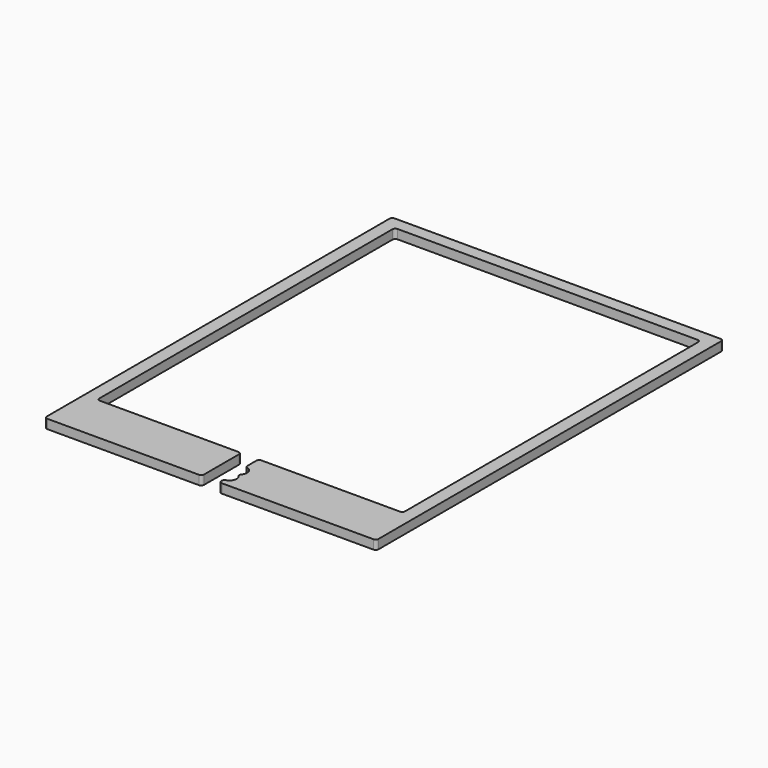
from build123d import *

# Parameters (mm, degrees)
F1_DEPTH = 6.35
F2_R     = 2


# Not quite as in the source:
# - a length typed as a fraction of an inch, garbled in the dataset ("3 / 203.2 mm" for 3/8 in), is restored


with BuildPart() as f1:
    # F0 (on Top) → F1 (new body)
    with BuildSketch(Plane.XY):
        with BuildLine():
            Line((115, -150.5), (115, 150.5))
            Line((115, 150.5), (-115, 150.5))
            Line((-115, 150.5), (-115, -150.5))
            Line((-115, -150.5), (-6, -150.5))
            Line((-6, -150.5), (-6, -116.2))
            Line((-6, -116.2), (-106, -116.2))
            Line((-106, -116.2), (-106, 141.8))
            Line((-106, 141.8), (106, 141.8))
            Line((106, 141.8), (106, -116.2))
            Line((106, -116.2), (6, -116.2))
            Line((6, -116.2), (6, -127.5))
            ThreePointArc((6, -127.5), (10.8733971724, -131.3819660113), (8.1794494718, -137))
            ThreePointArc((8.1794494718, -137), (10.8733971724, -142.6180339887), (6, -146.5))
            Line((6, -146.5), (6, -150.5))
            Line((6, -150.5), (115, -150.5))
        make_face()
    extrude(amount=F1_DEPTH)

    # F2
    f2_edges = [f1.edges().sort_by_distance(p)[0] for p in [
        (115, -150.5, 3.175),
        (115, 150.5, 3.175),
        (6, -116.2, 3.175),
        (-6, -116.2, 3.175),
        (-6, -150.5, 3.175),
        (-106, -116.2, 3.175),
        (-115, 150.5, 3.175),
        (6, -127.5, 3.175),
        (8.179449, -137, 3.175),
        (6, -146.5, 3.175),
        (-115, -150.5, 3.175),
        (106, 141.8, 3.175),
        (106, -116.2, 3.175),
        (-106, 141.8, 3.175),
        (6, -150.5, 3.175),
    ]]
    fillet(f2_edges, radius=F2_R)


solid = f1.part
